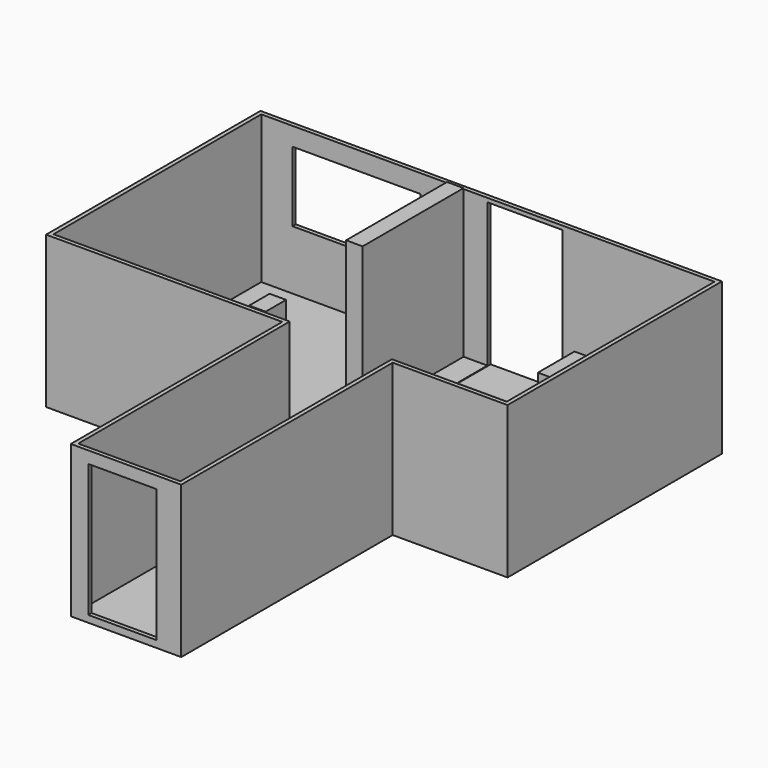
from build123d import *

# Parameters (mm, degrees)
F1_DEPTH  = 92
F2_T      = -2.5
F4_E13_W  = 76.4850056171
F4_E13_H  = 90
F5_DEPTH  = 10
F7_E14_W  = 15.5262811482
F7_E14_H  = 90
F8_DEPTH  = 10
F9_W      = 41.4156280458
F9_H      = 80.5949582718
F10_DEPTH = 25
F12_W     = 45.5428082496
F12_H     = 87.5177572016
F13_DEPTH = 25
F14_W     = 77.7512546629
F14_H     = 42.4544923007
F15_DEPTH = 25
F16_W     = 35.3893190622
F16_H     = 128.1821280718
F17_DEPTH = 25


with BuildPart() as f1:
    # F0 (on Top) → F1 (new body)
    with BuildSketch(Plane.XY):
        Polygon((22.0979973674, 49.8246140778), (22.0979973674, -110.3982031345), (89.0265107155, -110.3982031345), (89.0265107155, 49.8246140778), (158.6511880159, 49.8246140778), (158.6511880159, 212.2613489628), (0, 212.2613489628), (-121.0884749889, 212.2613489628), (-121.0884749889, 49.8246140778), (0, 49.8246140778), align=None)
    extrude(amount=F1_DEPTH)

    # F2
    f2_openings = [f1.faces().sort_by_distance(p)[0] for p in [
        (25.804053, 100.239761, 92),
    ]]
    offset(amount=F2_T, openings=f2_openings, kind=Kind.INTERSECTION)

    # F4_E13 (on explicit) → F5 (join)
    with BuildSketch(Plane(origin=(4.0378416888, 209.7613489628, 2.5), x_dir=(0, -1, 0), z_dir=(-1, 0, 0))):
        with Locations((38.2425028086, 45)):
            Rectangle(F4_E13_W, F4_E13_H)
    extrude(amount=F5_DEPTH)

    # F7_E14 (on explicit) → F8 (join)
    with BuildSketch(Plane(origin=(0, 52.3246140778, 2.5), x_dir=(0, 1, 0), z_dir=(1, 0, 0))):
        with Locations((7.7631405741, 45)):
            Rectangle(F7_E14_W, F7_E14_H)
    extrude(amount=F8_DEPTH)

    # F9 (on face) → F10 (cut)
    with BuildSketch(Plane.XZ.offset(110.3982031345)):
        with Locations((53.3959884197, 44.4829904009)):
            Rectangle(F9_W, F9_H)
    extrude(amount=-F10_DEPTH, mode=Mode.SUBTRACT)

    # F12 (on face) → F13 (cut)
    with BuildSketch(Plane(origin=(0, 212.2613489628, 0), x_dir=(-1, 0, 0), z_dir=(0, 1, 0))):
        with Locations((-41.2379493937, 45.8978245733)):
            Rectangle(F12_W, F12_H)
    extrude(amount=-F13_DEPTH, mode=Mode.SUBTRACT)

    # F14 (on face) → F15 (cut)
    with BuildSketch(Plane.XZ.offset(-209.7613489628)):
        with Locations((-60.8778791502, 59.6545059234)):
            Rectangle(F14_W, F14_H)
    extrude(amount=-F15_DEPTH, mode=Mode.SUBTRACT)

    # F16 (on face) → F17 (join)
    with BuildSketch(Plane.XY.offset(2.5)):
        Polygon((155.4546654224, 209.2887163162), (71.6699585319, 209.2887163162), (71.6699585319, 181.543186307), (120.0653463602, 181.543186307), (155.4546654224, 181.543186307), align=None)
        with Locations((137.7600058913, 117.4521222711)):
            Rectangle(F16_W, F16_H)
    extrude(amount=F17_DEPTH)


solid = f1.part
